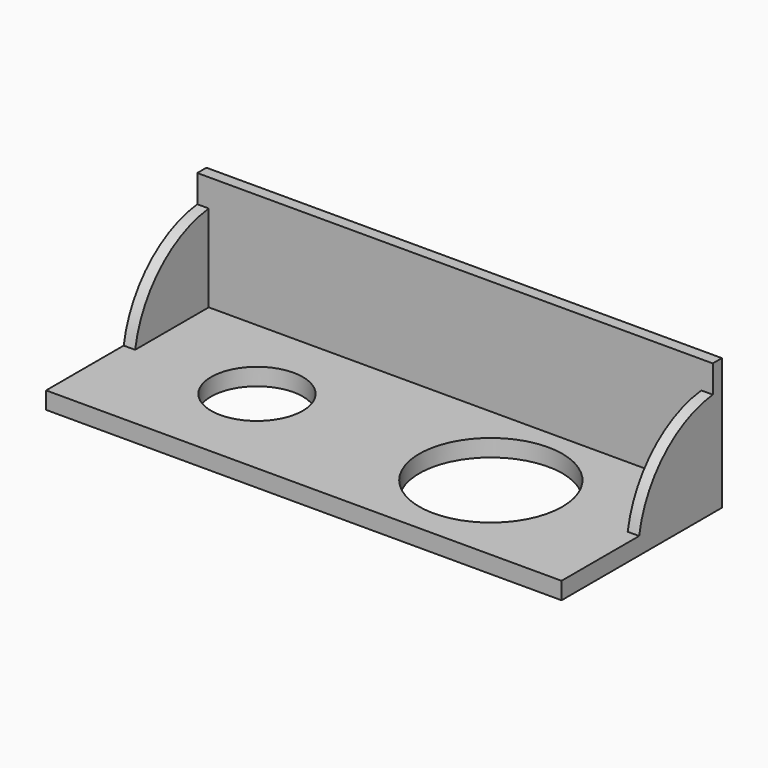
from build123d import *

# Parameters (mm, degrees)
F0_W          = 90
F0_H          = 35
F1_DEPTH      = 3
F2_W          = 90
F2_H          = 23
F3_DEPTH      = 2
F5_DEPTH      = 45
F5_DEPTH_BACK = 45
F7_START      = 3
F6_W          = 86
F6_H          = 33
F7_DEPTH      = 32.9
F8_R          = 12.5
F8_R_2        = 8
F9_DEPTH      = 3


with BuildPart() as f1:
    # F0 (on Top) → F1 (new body)
    with BuildSketch(Plane.XY):
        with Locations((0, -17.5)):
            Rectangle(F0_W, F0_H)
    extrude(amount=F1_DEPTH)

    # F2 (on Front) → F3 (join)
    with BuildSketch(Plane.XZ):
        with Locations((0, 11.5)):
            Rectangle(F2_W, F2_H)
    extrude(amount=F3_DEPTH)

    # F4 (on Right) → F5 (join, two sides)
    with BuildSketch(Plane.YZ) as f5_sk:
        with BuildLine():
            Line((-18.3083641247, 0), (0, 0))
            Line((0, 0), (0, 18.3083641247))
            ThreePointArc((0, 18.3083641247), (-12.945968425, 12.945968425), (-18.3083641247, 0))
        make_face()
    extrude(amount=F5_DEPTH)
    extrude(f5_sk.sketch, amount=-F5_DEPTH_BACK)

    # F6 (on Top) → F7 (cut)
    with BuildSketch(Plane.XY.offset(F7_START)):
        with Locations((0, -18.5)):
            Rectangle(F6_W, F6_H)
    extrude(amount=F7_DEPTH, mode=Mode.SUBTRACT)

    # F8 (on Top) → F9 (cut)
    with BuildSketch(Plane.XY):
        with Locations((18.9312342554, -17.8462527692)):
            Circle(F8_R)
        with Locations((-21.9019707292, -17.8462527692)):
            Circle(F8_R_2)
    extrude(amount=F9_DEPTH, mode=Mode.SUBTRACT)


solid = f1.part
